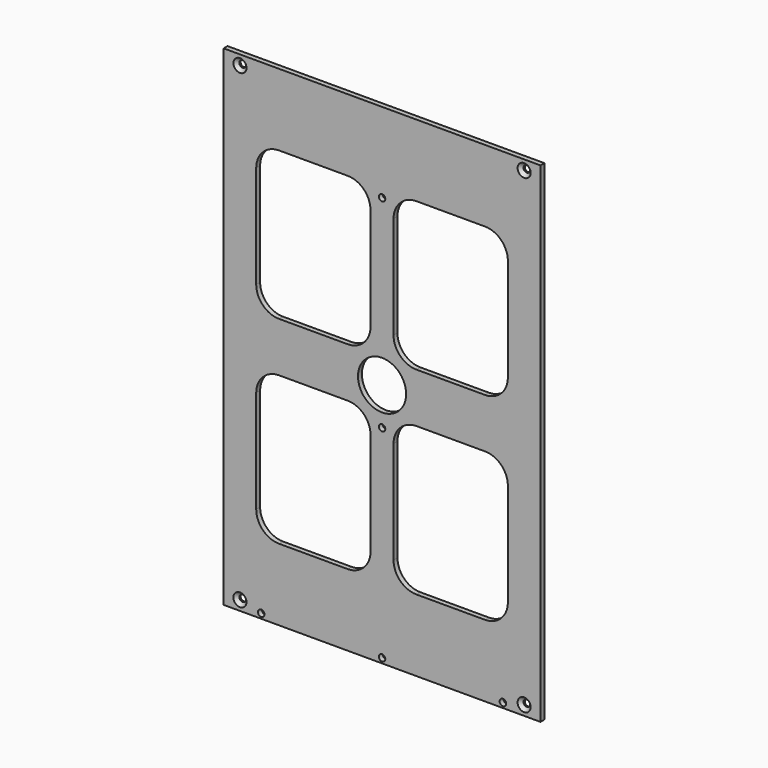
from build123d import *

# Parameters (mm, degrees)
F0_W           = 97
F0_H           = 150
F0_R           = 7.367785
F1_DEPTH       = 1.5
F3_D           = 2
F3_CSINK_D     = 4
F3_CSINK_ANGLE = 90
F5_D           = 2


# Not quite as in the source:
# - a feature names something its author has since deleted; it is built from what else it names


with BuildPart() as f1:
    # F0 (on Front) → F1 (new body)
    with BuildSketch(Plane.XZ):
        Rectangle(F0_W, F0_H)
        with BuildLine():
            Line((-31.5249225795, -7.60684), (-10.5249225795, -7.60684))
            ThreePointArc((-10.5249225795, -7.60684), (-5.5751751112, -9.6570925317), (-3.5249225795, -14.60684))
            Line((-3.5249225795, -14.60684), (-3.5249225795, -46))
            ThreePointArc((-3.5249225795, -46), (-5.5751751112, -50.9497474683), (-10.5249225795, -53))
            Line((-10.5249225795, -53), (-31.5249225795, -53))
            ThreePointArc((-31.5249225795, -53), (-36.4746700478, -50.9497474683), (-38.5249225795, -46))
            Line((-38.5249225795, -46), (-38.5249225795, -14.60684))
            ThreePointArc((-38.5249225795, -14.60684), (-36.4746700478, -9.6570925317), (-31.5249225795, -7.60684))
        make_face(mode=Mode.SUBTRACT)
        with BuildLine():
            ThreePointArc((38.5249225795, -46), (36.4746700478, -50.9497474683), (31.5249225795, -53))
            Line((31.5249225795, -53), (10.5249225795, -53))
            ThreePointArc((10.5249225795, -53), (5.5751751112, -50.9497474683), (3.5249225795, -46))
            Line((3.5249225795, -46), (3.5249225795, -14.60684))
            ThreePointArc((3.5249225795, -14.60684), (5.5751751112, -9.6570925317), (10.5249225795, -7.60684))
            Line((10.5249225795, -7.60684), (31.5249225795, -7.60684))
            ThreePointArc((31.5249225795, -7.60684), (36.4746700478, -9.6570925317), (38.5249225795, -14.60684))
            Line((38.5249225795, -14.60684), (38.5249225795, -46))
        make_face(mode=Mode.SUBTRACT)
        with BuildLine():
            ThreePointArc((-3.5249225795, 14.60684), (-5.5751751112, 9.6570925317), (-10.5249225795, 7.60684))
            Line((-10.5249225795, 7.60684), (-31.5249225795, 7.60684))
            ThreePointArc((-31.5249225795, 7.60684), (-36.4746700478, 9.6570925317), (-38.5249225795, 14.60684))
            Line((-38.5249225795, 14.60684), (-38.5249225795, 46))
            ThreePointArc((-38.5249225795, 46), (-36.4746700478, 50.9497474683), (-31.5249225795, 53))
            Line((-31.5249225795, 53), (-10.5249225795, 53))
            ThreePointArc((-10.5249225795, 53), (-5.5751751112, 50.9497474683), (-3.5249225795, 46))
            Line((-3.5249225795, 46), (-3.5249225795, 14.60684))
        make_face(mode=Mode.SUBTRACT)
        Circle(F0_R, mode=Mode.SUBTRACT)
        with BuildLine():
            ThreePointArc((10.5249225795, 7.60684), (5.5751751112, 9.6570925317), (3.5249225795, 14.60684))
            Line((3.5249225795, 14.60684), (3.5249225795, 46))
            ThreePointArc((3.5249225795, 46), (5.5751751112, 50.9497474683), (10.5249225795, 53))
            Line((10.5249225795, 53), (31.5249225795, 53))
            ThreePointArc((31.5249225795, 53), (36.4746700478, 50.9497474683), (38.5249225795, 46))
            Line((38.5249225795, 46), (38.5249225795, 14.60684))
            ThreePointArc((38.5249225795, 14.60684), (36.4746700478, 9.6570925317), (31.5249225795, 7.60684))
            Line((31.5249225795, 7.60684), (10.5249225795, 7.60684))
        make_face(mode=Mode.SUBTRACT)
    extrude(amount=F1_DEPTH)

    # F3 (through all)
    with Locations(Plane.XZ.offset(1.5)):
        with Locations((-43.5, -72), (43.5, -72), (43.5, 72), (-43.5, 72)):
            CounterSinkHole(F3_D / 2, F3_CSINK_D / 2, counter_sink_angle=F3_CSINK_ANGLE)

    # F5 (through all)
    with Locations(Plane.XZ.offset(1.5)):
        with Locations((-37, -73.5), (0, -73.5), (37, -73.5), (0, -11.5), (0, 50.5)):
            Hole(F5_D / 2)


solid = f1.part
